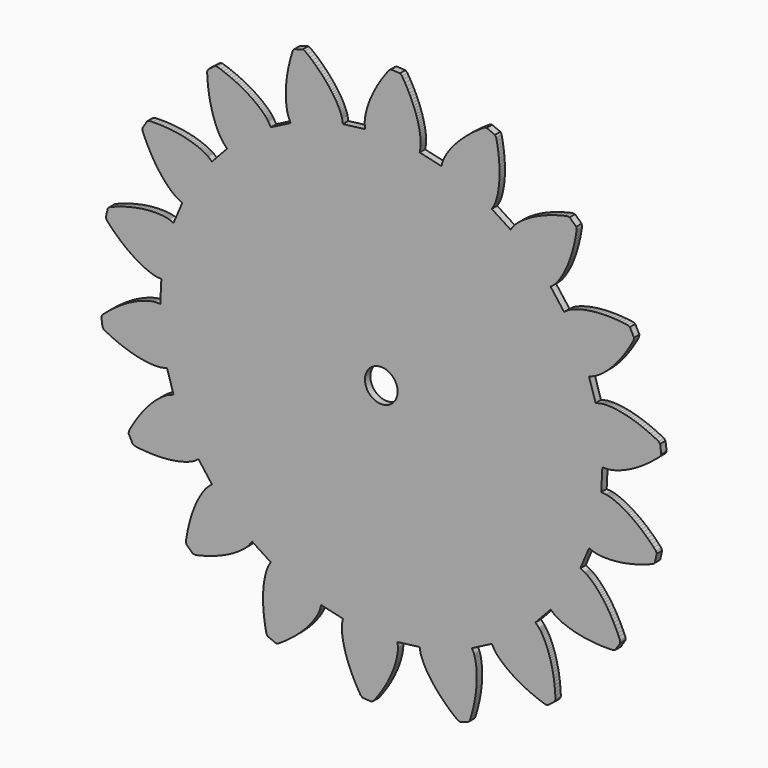
from build123d import *

# Parameters (mm, degrees)
F0_R     = 3.8384091464
F1_DEPTH = 1.5875


# Not quite as in the source:
# - a length typed as a fraction of an inch, garbled in the dataset ("3 / 203.2 mm" for 3/8 in), is restored


with BuildPart() as f1:
    # F0 (on Front) → F1 (new body)
    with BuildSketch(Plane.XZ):
        Polygon((51.660171, -5.23113), (51.924585, 0), (53.050313, 0), (53.079269, 0.00127), (53.126259, 0.002794), (53.193569, 0.008128), (53.281961, 0.014986), (53.389403, 0.025908), (53.516149, 0.042672), (53.662199, 0.0635), (53.827553, 0.090932), (54.010941, 0.124206), (54.214903, 0.166878), (54.436899, 0.216154), (54.676421, 0.275336), (54.935755, 0.343154), (55.211091, 0.42291), (55.504715, 0.513842), (55.814849, 0.61595), (56.142763, 0.73025), (56.487187, 0.85852), (56.847105, 1.000506), (57.221755, 1.157478), (57.613169, 1.329944), (58.018299, 1.518666), (58.436891, 1.722628), (58.871231, 1.94437), (59.317763, 2.183892), (59.776487, 2.441956), (60.247911, 2.718816), (60.730003, 3.01498), (61.223525, 3.331972), (61.727969, 3.669538), (62.242065, 4.027932), (62.764035, 4.40817), (63.296165, 4.809236), (63.834899, 5.23367), (64.380491, 5.681472), (64.933449, 6.152642), (65.491487, 6.647688), (65.759965, 7.135622), (65.498091, 9.23417), (65.119377, 9.64057), (64.456437, 9.983978), (63.804419, 10.305034), (63.165355, 10.603992), (62.537975, 10.8839), (61.924819, 11.142726), (61.324109, 11.382756), (60.738385, 11.604498), (60.166631, 11.806936), (59.611387, 11.992864), (59.069605, 12.161266), (58.544587, 12.31392), (58.037603, 12.451842), (57.545605, 12.574778), (57.069863, 12.681966), (56.613933, 12.778486), (56.174259, 12.861036), (55.754143, 12.931394), (55.351553, 12.9921), (54.967505, 13.04036), (54.601999, 13.080238), (54.257575, 13.111988), (53.930931, 13.133832), (53.623591, 13.150342), (53.336825, 13.158978), (53.069871, 13.163042), (52.821459, 13.160248), (52.594383, 13.15466), (52.387627, 13.145008), (52.200175, 13.132816), (52.033297, 13.1191), (51.887247, 13.102336), (51.760755, 13.08735), (51.653059, 13.07211), (51.566191, 13.05687), (51.499897, 13.045694), (51.453415, 13.036042), (51.425475, 13.029438), (50.334291, 12.753594), (48.793781, 17.758664), (49.852199, 18.144744), (49.876837, 18.154142), (49.922303, 18.1737), (49.984533, 18.201132), (50.062765, 18.238216), (50.160809, 18.285206), (50.273585, 18.342864), (50.403125, 18.413222), (50.549175, 18.494756), (50.711735, 18.589498), (50.888265, 18.698464), (51.079781, 18.8214), (51.285013, 18.958814), (51.504215, 19.111976), (51.737133, 19.27987), (51.982497, 19.466306), (52.238783, 19.668744), (52.507515, 19.889216), (52.785899, 20.126198), (53.076475, 20.383754), (53.375687, 20.659598), (53.683027, 20.954238), (53.999765, 21.26996), (54.323615, 21.606256), (54.655847, 21.961856), (54.993413, 22.34057), (55.336313, 22.740366), (55.683785, 23.160482), (56.036591, 23.60422), (56.392191, 24.071326), (56.750331, 24.560784), (57.110249, 25.073356), (57.472453, 25.608026), (57.833641, 26.167588), (58.194575, 26.751788), (58.555509, 27.358086), (58.913903, 27.9908), (59.268233, 28.646628), (59.353577, 29.196538), (58.388885, 31.078932), (57.894093, 31.331154), (57.154191, 31.42742), (56.432069, 31.50616), (55.729505, 31.567882), (55.044213, 31.616142), (54.378987, 31.650686), (53.732557, 31.669736), (53.106955, 31.678372), (52.500403, 31.672784), (51.913409, 31.657544), (51.348513, 31.631382), (50.802921, 31.595822), (50.277903, 31.550356), (49.774983, 31.497778), (49.291113, 31.437072), (48.829341, 31.371032), (48.388397, 31.29788), (47.968281, 31.220664), (47.570009, 31.139638), (47.192311, 31.053786), (46.835441, 30.967172), (46.500669, 30.87751), (46.186471, 30.787848), (45.892847, 30.69717), (45.619797, 30.607508), (45.368083, 30.51937), (45.134911, 30.432756), (44.924091, 30.349698), (44.732575, 30.269942), (44.560363, 30.19425), (44.408725, 30.123892), (44.276391, 30.059122), (44.162091, 30.00121), (44.066841, 29.950156), (43.991149, 29.907484), (43.931713, 29.873194), (43.891835, 29.846778), (43.868721, 29.832808), (42.937049, 29.199332), (39.777035, 33.375854), (40.639619, 34.10077), (40.660447, 34.118804), (40.694737, 34.152078), (40.744521, 34.19856), (40.806497, 34.260536), (40.880919, 34.338006), (40.967787, 34.431732), (41.066847, 34.541714), (41.175813, 34.66846), (41.294431, 34.813494), (41.423971, 34.976054), (41.561893, 35.156394), (41.707943, 35.356292), (41.862121, 35.575494), (42.021887, 35.812476), (42.188765, 36.071556), (42.360977, 36.348416), (42.538777, 36.647628), (42.719371, 36.96716), (42.903775, 37.30752), (43.089957, 37.668454), (43.278933, 38.051486), (43.468925, 38.45687), (43.659171, 38.882828), (43.847893, 39.330376), (44.035091, 39.8018), (44.221527, 40.293798), (44.404661, 40.809164), (44.583731, 41.346628), (44.758737, 41.905936), (44.928155, 42.488866), (45.090715, 43.093894), (45.246671, 43.72102), (45.395515, 44.369736), (45.535977, 45.042582), (45.666787, 45.735748), (45.786675, 46.452282), (45.897165, 47.189644), (45.788199, 47.735236), (44.237783, 49.175416), (43.686603, 49.242726), (42.958893, 49.078642), (42.253281, 48.90643), (41.571291, 48.724566), (40.911399, 48.535844), (40.274621, 48.34001), (39.659941, 48.137572), (39.070153, 47.930816), (38.501193, 47.718726), (37.955347, 47.503588), (37.432869, 47.28591), (36.932743, 47.065438), (36.454715, 46.843442), (36.000055, 46.6217), (35.565715, 46.399704), (35.154997, 46.179232), (34.765107, 45.960284), (34.397315, 45.743876), (34.051113, 45.531532), (33.724977, 45.322236), (33.420177, 45.118528), (33.134935, 44.9199), (32.870521, 44.728384), (32.624903, 44.542456), (32.399097, 44.364656), (32.192341, 44.194984), (32.005143, 44.034964), (31.833947, 43.88358), (31.682563, 43.742864), (31.546165, 43.613578), (31.427547, 43.49496), (31.325693, 43.388788), (31.238825, 43.296332), (31.165927, 43.215306), (31.109285, 43.149266), (31.066613, 43.096688), (31.036387, 43.059604), (31.019877, 43.037506), (30.361255, 42.123614), (25.962483, 44.96816), (26.525855, 45.94352), (26.538555, 45.968666), (26.560399, 46.009814), (26.590625, 46.072044), (26.627709, 46.150276), (26.671905, 46.249844), (26.721435, 46.366938), (26.775283, 46.504606), (26.834465, 46.660308), (26.897965, 46.838108), (26.962735, 47.033688), (27.031569, 47.251366), (27.100403, 47.488348), (27.169491, 47.746158), (27.239849, 48.026066), (27.307159, 48.32477), (27.374977, 48.64481), (27.437969, 48.986186), (27.500199, 49.348898), (27.556587, 49.73066), (27.607641, 50.134266), (27.654631, 50.5587), (27.694509, 51.003708), (27.726259, 51.469544), (27.750897, 51.955954), (27.767661, 52.461922), (27.773249, 52.98821), (27.768931, 53.535326), (27.753691, 54.101492), (27.726259, 54.68747), (27.686127, 55.292244), (27.632533, 55.916576), (27.564969, 56.559958), (27.482165, 57.220104), (27.384375, 57.899554), (27.270075, 58.597038), (27.137741, 59.310778), (26.988897, 60.041028), (26.701115, 60.517786), (24.750903, 61.340492), (24.209375, 61.215016), (23.582503, 60.81268), (22.978999, 60.40882), (22.398609, 60.005214), (21.843365, 59.601354), (21.312759, 59.199272), (20.804505, 58.799476), (20.320635, 58.402728), (19.858863, 58.010044), (19.419443, 57.62117), (19.003137, 57.236614), (18.607659, 56.85917), (18.235549, 56.48706), (17.882743, 56.121808), (17.552035, 55.766208), (17.240631, 55.41772), (16.950055, 55.078884), (16.677005, 54.749192), (16.425037, 54.431184), (16.189325, 54.123844), (15.972663, 53.827426), (15.773019, 53.543454), (15.589631, 53.272182), (15.423007, 53.014372), (15.271369, 52.770532), (15.136241, 52.540408), (15.013813, 52.32527), (14.904847, 52.125626), (14.809597, 51.940714), (14.727047, 51.77282), (14.655419, 51.621182), (14.596237, 51.486054), (14.546453, 51.36896), (14.506575, 51.268376), (14.474825, 51.18735), (14.452981, 51.122326), (14.437741, 51.07686), (14.429359, 51.050698), (14.122019, 49.967642), (9.016619, 51.136042), (9.212199, 52.244244), (9.216263, 52.2732), (9.222105, 52.319936), (9.230233, 52.3875), (9.237091, 52.474114), (9.245219, 52.58181), (9.251061, 52.709826), (9.256141, 52.8574), (9.257665, 53.025548), (9.256141, 53.213), (9.251061, 53.419756), (9.239631, 53.646832), (9.223375, 53.89372), (9.201277, 54.159404), (9.170797, 54.44617), (9.132443, 54.750716), (9.085453, 55.074566), (9.029065, 55.41645), (8.962771, 55.777384), (8.885809, 56.156606), (8.796147, 56.553354), (8.694293, 56.967882), (8.579485, 57.400698), (8.451469, 57.8485), (8.308213, 58.314336), (8.149971, 58.795158), (7.974457, 59.292744), (7.784465, 59.803792), (7.575169, 60.331858), (7.349109, 60.872116), (7.105269, 61.42736), (6.842125, 61.99505), (6.558153, 62.57671), (6.254877, 63.169292), (5.930011, 63.774066), (5.583809, 64.390016), (5.215763, 65.015872), (4.826127, 65.651126), (4.391787, 65.999614), (2.279269, 66.10731), (1.813687, 65.804034), (1.360043, 65.210182), (0.931799, 64.624458), (0.524891, 64.047116), (0.141859, 63.478156), (-0.220345, 62.918594), (-0.560959, 62.369954), (-0.880491, 61.83122), (-1.179703, 61.303154), (-1.459357, 60.788042), (-1.719707, 60.283598), (-1.961007, 59.794394), (-2.184019, 59.317636), (-2.390775, 58.854594), (-2.579497, 58.405522), (-2.753487, 57.972706), (-2.910459, 57.554876), (-3.053715, 57.152794), (-3.181985, 56.766714), (-3.297809, 56.397398), (-3.401187, 56.044592), (-3.490595, 55.70982), (-3.570351, 55.391558), (-3.639185, 55.0926), (-3.697097, 54.811422), (-3.746881, 54.548278), (-3.788029, 54.304438), (-3.821303, 54.079648), (-3.847465, 53.874416), (-3.868039, 53.688488), (-3.883279, 53.520086), (-3.894201, 53.374036), (-3.899789, 53.24602), (-3.903853, 53.138578), (-3.905123, 53.050186), (-3.903853, 52.982876), (-3.902329, 52.934616), (-3.901313, 52.90693), (-3.818509, 51.783742), (-9.016619, 51.136042), (-9.211945, 52.244244), (-9.217787, 52.271676), (-9.228709, 52.318666), (-9.245219, 52.384706), (-9.267317, 52.47005), (-9.296273, 52.573428), (-9.334881, 52.694586), (-9.380347, 52.835556), (-9.436735, 52.993798), (-9.501759, 53.168804), (-9.577197, 53.361844), (-9.665335, 53.570886), (-9.764903, 53.79847), (-9.877679, 54.041294), (-10.004425, 54.29885), (-10.143617, 54.571392), (-10.297795, 54.861206), (-10.468991, 55.162704), (-10.654919, 55.47995), (-10.857357, 55.809134), (-11.076559, 56.152288), (-11.313541, 56.506364), (-11.570081, 56.872886), (-11.844147, 57.250584), (-12.137517, 57.639204), (-12.451969, 58.037476), (-12.785217, 58.443876), (-13.139547, 58.860182), (-13.515467, 59.284616), (-13.912469, 59.714638), (-14.332839, 60.152788), (-14.775307, 60.596526), (-15.239619, 61.045598), (-15.727553, 61.498988), (-16.240125, 61.956442), (-16.774795, 62.416944), (-17.335881, 62.878208), (-17.920081, 63.343028), (-18.444845, 63.522098), (-20.468209, 62.899036), (-20.802981, 62.455298), (-21.024723, 61.743082), (-21.227415, 61.045598), (-21.411819, 60.363354), (-21.577173, 59.698128), (-21.726017, 59.048904), (-21.858351, 58.416444), (-21.974175, 57.800494), (-22.074759, 57.20207), (-22.161373, 56.622188), (-22.234525, 56.061356), (-22.293707, 55.517034), (-22.340697, 54.993286), (-22.375241, 54.487572), (-22.399879, 54.000908), (-22.415119, 53.535326), (-22.420707, 53.08727), (-22.416389, 52.661566), (-22.405467, 52.253642), (-22.387687, 51.867816), (-22.364319, 51.501294), (-22.333839, 51.1556), (-22.300819, 50.830226), (-22.261957, 50.52568), (-22.220809, 50.241708), (-22.178137, 49.977294), (-22.132417, 49.73447), (-22.086951, 49.511458), (-22.041485, 49.308766), (-21.997543, 49.127156), (-21.954617, 48.964342), (-21.913469, 48.82261), (-21.876385, 48.701198), (-21.843365, 48.599344), (-21.812885, 48.515016), (-21.789517, 48.45177), (-21.773007, 48.407828), (-21.761831, 48.381666), (-21.300313, 47.354744), (-25.962229, 44.96816), (-26.525601, 45.94352), (-26.539317, 45.967142), (-26.565987, 46.00702), (-26.604341, 46.063408), (-26.654125, 46.135036), (-26.717117, 46.221904), (-26.794587, 46.324266), (-26.885519, 46.439836), (-26.991691, 46.5709), (-27.114119, 46.712632), (-27.250517, 46.868334), (-27.405203, 47.034958), (-27.575891, 47.214282), (-27.764613, 47.403004), (-27.971369, 47.603156), (-28.197429, 47.810928), (-28.441269, 48.029876), (-28.704413, 48.255936), (-28.987115, 48.488854), (-29.290137, 48.730154), (-29.613987, 48.976788), (-29.958665, 49.22901), (-30.323663, 49.485042), (-30.711013, 49.74717), (-31.120207, 50.011838), (-31.550229, 50.277776), (-32.003619, 50.546254), (-32.478853, 50.81651), (-32.976439, 51.086766), (-33.497393, 51.355244), (-34.041715, 51.622706), (-34.609405, 51.888644), (-35.199193, 52.151788), (-35.813873, 52.410614), (-36.450397, 52.665884), (-37.110543, 52.915058), (-37.795327, 53.157882), (-38.503733, 53.393594), (-39.058977, 53.382164), (-40.7471626, 52.104798), (-40.9083764, 51.572922), (-40.8739594, 50.828956), (-40.8257248, 50.103786), (-40.7664666, 49.399698), (-40.694737, 48.717708), (-40.612187, 48.056292), (-40.519731, 47.41672), (-40.417877, 46.7995), (-40.308911, 46.202854), (-40.190547, 45.628306), (-40.066341, 45.075348), (-39.936801, 44.54525), (-39.801927, 44.034964), (-39.662735, 43.548554), (-39.519225, 43.082972), (-39.373175, 42.640504), (-39.224331, 42.218864), (-39.075487, 41.817798), (-38.926643, 41.440354), (-38.778053, 41.08196), (-38.629209, 40.747188), (-38.483159, 40.431466), (-38.339649, 40.137842), (-38.200457, 39.863776), (-38.064059, 39.611554), (-37.933249, 39.378636), (-37.807773, 39.165276), (-37.689409, 38.970966), (-37.577649, 38.79596), (-37.473001, 38.640004), (-37.377751, 38.50386), (-37.291137, 38.383972), (-37.213921, 38.281864), (-37.147627, 38.197536), (-37.091239, 38.128956), (-37.047043, 38.078156), (-37.015547, 38.042088), (-36.997513, 38.02126), (-36.212145, 37.213794), (-39.777035, 33.375854), (-40.639619, 34.10077), (-40.661717, 34.117534), (-40.699055, 34.146236), (-40.754046, 34.186114), (-40.8257248, 34.237422), (-40.9153106, 34.298128), (-41.0228034, 34.366708), (-41.1481778, 34.444178), (-41.29151, 34.529522), (-41.455467, 34.621978), (-41.6373564, 34.721038), (-41.8399722, 34.825686), (-42.0618158, 34.934398), (-42.3029888, 35.047682), (-42.5661836, 35.164776), (-42.848657, 35.284664), (-43.1532284, 35.405822), (-43.4770784, 35.528504), (-43.8229756, 35.651186), (-44.1908692, 35.773614), (-44.5794892, 35.895026), (-44.9887594, 36.013644), (-45.4201022, 36.130738), (-45.8734922, 36.243514), (-46.347507, 36.35121), (-46.8436198, 36.454588), (-47.3617544, 36.552378), (-47.9005392, 36.64331), (-48.4600504, 36.72586), (-49.0415834, 36.801806), (-49.6451636, 36.866576), (-50.2694194, 36.922964), (-50.9129538, 36.96716), (-51.5785354, 37.001704), (-52.2647926, 37.022278), (-52.9703538, 37.03066), (-53.6965906, 37.025072), (-54.442106, 37.004498), (-54.9616376, 36.803076), (-56.1109114, 35.026854), (-56.0805838, 34.47161), (-55.7939448, 33.784032), (-55.5004478, 33.118298), (-55.2041822, 32.478726), (-54.9023794, 31.861506), (-54.599205, 31.269178), (-54.293262, 30.698694), (-53.9873698, 30.152848), (-53.6800806, 29.63037), (-53.372766, 29.130244), (-53.0668484, 28.653486), (-52.7636486, 28.198826), (-52.4618458, 27.767534), (-52.1642086, 27.356816), (-51.8707116, 26.967942), (-51.5826756, 26.60142), (-51.2988306, 26.255726), (-51.0218182, 25.931876), (-50.75174, 25.62733), (-50.4898914, 25.342088), (-50.2363232, 25.07742), (-49.9910354, 24.830786), (-49.755425, 24.603456), (-49.530762, 24.395176), (-49.3171988, 24.20366), (-49.1146338, 24.028654), (-48.923067, 23.871682), (-48.7453178, 23.72995), (-48.5799384, 23.60422), (-48.4297228, 23.494238), (-48.2919278, 23.397464), (-48.1692966, 23.314914), (-48.0631754, 23.24481), (-47.9708464, 23.187914), (-47.8950528, 23.143972), (-47.8371916, 23.109682), (-47.7944688, 23.087584), (-47.7696784, 23.075138), (-46.755431, 22.584664), (-48.793527, 17.758664), (-49.8518688, 18.144744), (-49.8780308, 18.152872), (-49.9235222, 18.167858), (-49.9882922, 18.185892), (-50.0737378, 18.20926), (-50.178462, 18.235422), (-50.3024648, 18.263108), (-50.4471686, 18.29308), (-50.611151, 18.325084), (-50.797206, 18.35531), (-51.0011426, 18.385536), (-51.2271264, 18.414492), (-51.4738366, 18.442178), (-51.7398, 18.4658), (-52.0264136, 18.48612), (-52.3323312, 18.50136), (-52.660296, 18.511266), (-53.0061932, 18.515076), (-53.3741376, 18.512536), (-53.7613606, 18.50136), (-54.1678876, 18.483834), (-54.5936932, 18.454878), (-55.0388028, 18.416016), (-55.503191, 18.367756), (-55.9855116, 18.307304), (-56.4871108, 18.235422), (-57.006617, 18.150078), (-57.544081, 18.050764), (-58.0994266, 17.936464), (-58.6713076, 17.808194), (-59.2597494, 17.663414), (-59.8660728, 17.502378), (-60.4861884, 17.324578), (-61.124211, 17.128998), (-61.7760512, 16.91386), (-62.4416328, 16.679672), (-63.1223782, 16.426434), (-63.8155188, 16.15186), (-64.234441, 15.786608), (-64.7071096, 13.72362), (-64.4893808, 13.212572), (-63.9836414, 12.663932), (-63.4806706, 12.138914), (-62.9831862, 11.638788), (-62.489842, 11.162284), (-62.0006634, 10.708386), (-61.5197144, 10.277348), (-61.0443026, 9.869678), (-60.5771204, 9.483598), (-60.1168978, 9.1186), (-59.6676226, 8.775192), (-59.2266532, 8.451342), (-58.7953612, 8.149844), (-58.375042, 7.865872), (-57.9671434, 7.601204), (-57.5702684, 7.356094), (-57.1857886, 7.126986), (-56.8137294, 6.916166), (-56.4568086, 6.723634), (-56.1123084, 6.54558), (-55.7829466, 6.38302), (-55.4687486, 6.2357), (-55.171086, 6.103366), (-54.8872156, 5.983478), (-54.6212522, 5.875782), (-54.3704526, 5.78231), (-54.13756, 5.699506), (-53.9225998, 5.627878), (-53.724175, 5.565648), (-53.5436064, 5.513578), (-53.3823926, 5.469382), (-53.2391112, 5.433314), (-53.1150576, 5.404358), (-53.0089364, 5.382514), (-52.9221192, 5.366004), (-52.8559776, 5.355082), (-52.80914, 5.34797), (-52.7802094, 5.345176), (-51.6598408, 5.230876), (-51.9244326, 0), (-53.0502876, 0), (-53.0792182, -0.001524), (-53.1260812, -0.002794), (-53.1936198, -0.008128), (-53.2818086, -0.01524), (-53.389276, -0.026162), (-53.5160728, -0.042672), (-53.6621482, -0.0635), (-53.8275022, -0.091186), (-54.0107886, -0.124206), (-54.2147506, -0.166878), (-54.4365942, -0.216408), (-54.6763956, -0.27559), (-54.9354756, -0.343408), (-55.2110656, -0.423164), (-55.5045626, -0.514096), (-55.8146204, -0.61595), (-56.1426106, -0.73025), (-56.4871108, -0.858774), (-56.8467748, -1.000506), (-57.2216026, -1.157478), (-57.6129658, -1.329944), (-58.0180958, -1.518666), (-58.4370434, -1.722628), (-58.8711294, -1.944624), (-59.3176106, -2.184146), (-59.776487, -2.441956), (-60.2477586, -2.718816), (-60.7300792, -3.015234), (-61.2234488, -3.331972), (-61.7278166, -3.669792), (-62.241811, -4.028186), (-62.7640858, -4.408424), (-63.2960126, -4.80949), (-63.8348228, -5.233924), (-64.3805164, -5.681472), (-64.9331188, -6.152896), (-65.491233, -6.647942), (-65.7599396, -7.135622), (-65.4981164, -9.234424), (-65.1191484, -9.640824), (-64.45631, -9.983978), (-63.8044952, -10.305034), (-63.165101, -10.604246), (-62.5380766, -10.8839), (-61.9248698, -11.14298), (-61.3240328, -11.382756), (-60.738385, -11.604752), (-60.1664786, -11.80719), (-59.6111584, -11.993118), (-59.0695542, -12.16152), (-58.5445362, -12.314174), (-58.0373998, -12.452096), (-57.5454526, -12.574778), (-57.0700154, -12.68222), (-56.6139076, -12.77874), (-56.1743098, -12.86129), (-55.754016, -12.931394), (-55.3516038, -12.9921), (-54.9671494, -13.040614), (-54.6019482, -13.080492), (-54.2574734, -13.112242), (-53.9308548, -13.134086), (-53.6235656, -13.150596), (-53.3369266, -13.158978), (-53.0695916, -13.163042), (-52.8215606, -13.160502), (-52.5941544, -13.154914), (-52.3874492, -13.145262), (-52.2000226, -13.13307), (-52.033297, -13.118846), (-51.8872216, -13.10259), (-51.7604756, -13.08735), (-51.6529828, -13.072364), (-51.5661656, -13.057124), (-51.4999986, -13.045694), (-51.453161, -13.036296), (-51.4255766, -13.029692), (-50.3341894, -12.753594), (-48.793527, -17.758918), (-49.8518688, -18.144744), (-49.8766592, -18.154396), (-49.9221506, -18.1737), (-49.984152, -18.201386), (-50.0627142, -18.23847), (-50.160555, -18.285206), (-50.2735342, -18.343118), (-50.4030742, -18.413222), (-50.549175, -18.494756), (-50.7117604, -18.589752), (-50.8881634, -18.698718), (-51.0797048, -18.8214), (-51.2850384, -18.959068), (-51.5041388, -19.11223), (-51.737006, -19.280124), (-51.9823192, -19.466306), (-52.2386306, -19.668744), (-52.5073372, -19.889216), (-52.7856958, -20.126452), (-53.076475, -20.384008), (-53.3755092, -20.659344), (-53.6828238, -20.954492), (-53.999765, -21.270214), (-54.323615, -21.606256), (-54.65572, -21.961856), (-54.9933114, -22.340824), (-55.3364654, -22.740366), (-55.6837088, -23.160736), (-56.0364894, -23.604474), (-56.3920386, -24.07158), (-56.750331, -24.560784), (-57.109995, -25.073356), (-57.4724276, -25.60828), (-57.8334632, -26.167842), (-58.1944988, -26.752042), (-58.5555598, -27.35834), (-58.9138522, -27.9908), (-59.2680044, -28.646628), (-59.35345, -29.196792), (-58.3888088, -31.078932), (-57.8941184, -31.331154), (-57.1540894, -31.427674), (-56.4319928, -31.50616), (-55.7292256, -31.568136), (-55.0442892, -31.616396), (-54.3787076, -31.65094), (-53.73243, -31.670244), (-53.1068026, -31.678372), (-52.5004538, -31.672784), (-51.9133836, -31.657798), (-51.3484114, -31.631636), (-50.8027178, -31.595822), (-50.2776744, -31.550356), (-49.7746782, -31.498032), (-49.2910114, -31.437326), (-48.8293664, -31.371032), (-48.388397, -31.298134), (-47.9681032, -31.220918), (-47.5698312, -31.139638), (-47.1922348, -31.05404), (-46.8353394, -30.967426), (-46.5004658, -30.877764), (-46.1862932, -30.788102), (-45.8927454, -30.697424), (-45.6198986, -30.607762), (-45.3677528, -30.519624), (-45.1348348, -30.432756), (-44.9239894, -30.349952), (-44.7324734, -30.270196), (-44.5602106, -30.19425), (-44.4086234, -30.124146), (-44.2763148, -30.059122), (-44.1619386, -30.001464), (-44.0668664, -29.950156), (-43.9910728, -29.907484), (-43.9317892, -29.873194), (-43.8918604, -29.846778), (-43.8684416, -29.833062), (-42.9368458, -29.199586), (-39.777035, -33.376108), (-40.639619, -34.101024), (-40.660447, -34.118804), (-40.694737, -34.152078), (-40.744521, -34.198814), (-40.8064208, -34.26079), (-40.8808428, -34.338006), (-40.96766, -34.431732), (-41.0668978, -34.541968), (-41.1757114, -34.668714), (-41.2942532, -34.813494), (-41.4237932, -34.976054), (-41.5615882, -35.156648), (-41.7076636, -35.356546), (-41.8620194, -35.575494), (-42.0218616, -35.812476), (-42.1885872, -36.071556), (-42.36085, -36.34867), (-42.5385992, -36.647628), (-42.719117, -36.967414), (-42.9038004, -37.307774), (-43.08983, -37.668708), (-43.2786282, -38.05174), (-43.4687726, -38.45687), (-43.6589678, -38.882828), (-43.847766, -39.33063), (-44.0351672, -39.802054), (-44.2212222, -40.293798), (-44.4044832, -40.8093164), (-44.5836294, -41.3467296), (-44.7586354, -41.9062408), (-44.928155, -42.4891454), (-45.0907404, -43.0940718), (-45.2464678, -43.7210962), (-45.3952864, -44.3701424), (-45.53585, -45.0426328), (-45.6667616, -45.7357734), (-45.786675, -46.4523836), (-45.896911, -47.1896186), (-45.7880466, -47.7353376), (-44.2377322, -49.1753652), (-43.6865014, -49.2428784), (-42.9589184, -49.0789214), (-42.2533572, -48.9066586), (-41.5712148, -48.7247692), (-40.911145, -48.5359456), (-40.274621, -48.340264), (-39.659941, -48.137699), (-39.070153, -47.9310192), (-38.500939, -47.7187768), (-37.955347, -47.5037912), (-37.432869, -47.2861132), (-36.932743, -47.0656158), (-36.454461, -46.8437468), (-35.999801, -46.6218524), (-35.565715, -46.3999834), (-35.154997, -46.1795114), (-34.765107, -45.9603856), (-34.397061, -45.7440792), (-34.051367, -45.5318368), (-33.724723, -45.3223884), (-33.420177, -45.1184264), (-33.134935, -44.9199762), (-32.870267, -44.7284602), (-32.624903, -44.5424052), (-32.399097, -44.3646306), (-32.192341, -44.1951364), (-32.004889, -44.0352942), (-31.833947, -43.883707), (-31.682563, -43.7431434), (-31.545911, -43.6136034), (-31.427547, -43.4951124), (-31.325439, -43.3889912), (-31.238825, -43.2966876), (-31.165673, -43.2153568), (-31.109285, -43.1492152), (-31.066359, -43.0968658), (-31.036133, -43.0596548), (-31.019623, -43.0376076), (-30.360747, -42.1239442), (-25.962229, -44.9682108), (-26.525601, -45.9438756), (-26.538301, -45.9686914), (-26.560145, -46.0100426), (-26.590625, -46.072044), (-26.627709, -46.1505808), (-26.671651, -46.2498186), (-26.721435, -46.366938), (-26.775029, -46.504733), (-26.834465, -46.6604604), (-26.897965, -46.8382096), (-26.962735, -47.0338912), (-27.031569, -47.2516454), (-27.100403, -47.4886528), (-27.169491, -47.7463358), (-27.239595, -48.0260914), (-27.307159, -48.3251256), (-27.374723, -48.6448354), (-27.437969, -48.9865924), (-27.499945, -49.3489996), (-27.556587, -49.7307108), (-27.607641, -50.1344946), (-27.654631, -50.5589286), (-27.694509, -51.0040128), (-27.726259, -51.469798), (-27.750897, -51.9562334), (-27.767407, -52.4619728), (-27.772995, -52.9883878), (-27.768931, -53.5354784), (-27.753691, -54.101873), (-27.726259, -54.6875208), (-27.685873, -55.292498), (-27.632279, -55.9167284), (-27.564969, -56.5602882), (-27.482165, -57.220358), (-27.384375, -57.8997318), (-27.270075, -58.597038), (-27.137741, -59.3108542), (-26.988897, -60.0412058), (-26.700607, -60.5180146), (-24.750903, -61.3406952), (-24.209375, -61.2152954), (-23.582503, -60.8129086), (-22.978745, -60.4091502), (-22.398609, -60.0053664), (-21.843365, -59.601608), (-21.312759, -59.1992212), (-20.804251, -58.799603), (-20.320635, -58.402728), (-19.858863, -58.0099678), (-19.419189, -57.6213478), (-19.003137, -57.2368934), (-18.607659, -56.8593224), (-18.235295, -56.4872378), (-17.882489, -56.122062), (-17.552035, -55.7665128), (-17.240631, -55.4178724), (-16.949801, -55.078884), (-16.676751, -54.7495476), (-16.425037, -54.4312348), (-16.189325, -54.1239202), (-15.972663, -53.8276292), (-15.773019, -53.5437334), (-15.589631, -53.2722836), (-15.423007, -53.0145752), (-15.271369, -52.770659), (-15.136241, -52.5405604), (-15.013813, -52.3255748), (-14.904847, -52.125753), (-14.809597, -51.9411204), (-14.727047, -51.7729724), (-14.655419, -51.6213852), (-14.596237, -51.4863334), (-14.546453, -51.369214), (-14.506575, -51.2686046), (-14.474825, -51.1873246), (-14.452981, -51.1225546), (-14.437741, -51.0770886), (-14.429359, -51.0508758), (-14.122019, -49.9677436), (-9.016619, -51.1363214), (-9.211945, -52.244244), (-9.216263, -52.2732254), (-9.221851, -52.320063), (-9.229979, -52.3875762), (-9.237091, -52.4743934), (-9.245219, -52.5818862), (-9.250807, -52.7100546), (-9.256141, -52.8574762), (-9.257665, -53.0256242), (-9.256141, -53.2130254), (-9.250807, -53.4197306), (-9.239631, -53.6471114), (-9.223375, -53.8937708), (-9.201023, -54.1597342), (-9.170797, -54.4463478), (-9.132189, -54.7509192), (-9.085453, -55.0747692), (-9.029065, -55.4165008), (-8.962517, -55.7775618), (-8.885301, -56.1565298), (-8.796147, -56.5534048), (-8.694293, -56.9681868), (-8.579485, -57.4008758), (-8.451469, -57.848754), (-8.308213, -58.3145392), (-8.149717, -58.7954882), (-7.974457, -59.2929218), (-7.784465, -59.804173), (-7.575169, -60.3319596), (-7.349109, -60.8721668), (-7.105269, -61.4275124), (-6.842125, -61.9952786), (-6.558153, -62.5767862), (-6.254623, -63.1693428), (-5.929757, -63.77432), (-5.583809, -64.3902954), (-5.215763, -65.0159228), (-4.825873, -65.6512022), (-4.391787, -65.9998426), (-2.279269, -66.1073354), (-1.813687, -65.804161), (-1.359789, -65.2102328), (-0.931545, -64.6245596), (-0.524891, -64.0471668), (-0.141859, -63.478029), (0.220599, -62.9185432), (0.560959, -62.3701064), (0.880491, -61.8312708), (1.179703, -61.3034842), (1.459357, -60.7880928), (1.719961, -60.2837504), (1.961261, -59.7945464), (2.184019, -59.3177376), (2.390775, -58.8546956), (2.580005, -58.4054712), (2.753487, -57.9727568), (2.910459, -57.5552062), (3.053715, -57.1528448), (3.181985, -56.7669934), (3.297809, -56.3976774), (3.401187, -56.0448968), (3.490849, -55.7100486), (3.570605, -55.3917104), (3.639185, -55.0926762), (3.697097, -54.811549), (3.746881, -54.5483542), (3.788283, -54.304438), (3.821303, -54.0798258), (3.847465, -53.8744668), (3.868293, -53.6884626), (3.883533, -53.5203146), (3.894455, -53.3742646), (3.900043, -53.2460962), (3.903853, -53.1386034), (3.905377, -53.0504146), (3.903853, -52.9829014), (3.902837, -52.9346668), (3.901313, -52.9071078), (3.818509, -51.7840214), (9.016619, -51.1363214), (9.212199, -52.244244), (9.217787, -52.2718284), (9.228709, -52.3186914), (9.245219, -52.384833), (9.267571, -52.4702786), (9.296527, -52.5736058), (9.334881, -52.6948908), (9.380347, -52.835429), (9.436735, -52.9938996), (9.501759, -53.1689056), (9.577197, -53.361844), (9.665335, -53.5713178), (9.764903, -53.7986986), (9.877933, -54.0412178), (10.004425, -54.2989262), (10.143871, -54.571773), (10.298049, -54.8611552), (10.468991, -55.162958), (10.654919, -55.4798992), (10.857357, -55.8092356), (11.076559, -56.1523896), (11.313541, -56.5065418), (11.570081, -56.8730892), (11.844147, -57.2506856), (12.137771, -57.6392802), (12.451969, -58.0375268), (12.785471, -58.4440792), (13.139547, -58.8602328), (13.515975, -59.2846668), (13.912977, -59.7146126), (14.333093, -60.1528134), (14.775307, -60.5965514), (15.239619, -61.0458012), (15.727553, -61.4991658), (16.240125, -61.9566706), (16.775049, -62.416944), (17.335881, -62.878589), (17.920081, -63.3429772), (18.445099, -63.5221234), (20.468209, -62.8992646), (20.802981, -62.455552), (21.024977, -61.743082), (21.227415, -61.0458012), (21.411819, -60.3636842), (21.577427, -59.6981026), (21.726271, -59.0490056), (21.858605, -58.4164948), (21.974175, -57.800494), (22.074759, -57.2024256), (22.161627, -56.6222896), (22.234525, -56.0614576), (22.293961, -55.5171102), (22.340697, -54.9934384), (22.375241, -54.487699), (22.400133, -54.0012636), (22.415119, -53.5354784), (22.420707, -53.0876256), (22.416643, -52.6617946), (22.405721, -52.2539214), (22.387687, -51.8680446), (22.364319, -51.5015226), (22.334093, -51.1556254), (22.300819, -50.8303784), (22.261957, -50.5258578), (22.220809, -50.2419874), (22.178137, -49.9773956), (22.132671, -49.7348764), (22.087205, -49.5116358), (22.041485, -49.3090454), (21.997543, -49.1271306), (21.954871, -48.9645452), (21.913469, -48.8225846), (21.876385, -48.7013504), (21.843365, -48.599344), (21.812885, -48.5152954), (21.789771, -48.451897), (21.773007, -48.4078026), (21.762085, -48.3816152), (21.300313, -47.354998), (25.962483, -44.9682108), (26.525855, -45.9438756), (26.539571, -45.9673198), (26.565987, -46.007274), (26.604341, -46.0637636), (26.654125, -46.135417), (26.717371, -46.2222342), (26.794587, -46.3242152), (26.885519, -46.439963), (26.991691, -46.5708746), (27.114119, -46.7128352), (27.250771, -46.8685626), (27.405203, -47.0352628), (27.575891, -47.214409), (27.764613, -47.4032326), (27.971369, -47.603029), (28.197683, -47.8111058), (28.441269, -48.0302062), (28.704413, -48.2562408), (28.987115, -48.489108), (29.290137, -48.7302556), (29.613987, -48.9769404), (29.958665, -49.229137), (30.323663, -49.485423), (30.711013, -49.7472462), (31.120207, -50.011838), (31.550483, -50.2778014), (32.003619, -50.546508), (32.478853, -50.816637), (32.976693, -51.0867152), (33.497393, -51.3554218), (34.041715, -51.6227568), (34.609405, -51.8887202), (35.199193, -52.1519404), (35.814127, -52.4110204), (36.450397, -52.6659602), (37.110543, -52.9153882), (37.795581, -53.1579074), (38.503987, -53.3935686), (39.059231, -53.3825196), (40.747315, -52.1050774), (40.908605, -51.5731506), (40.874061, -50.8290068), (40.826055, -50.104167), (40.766619, -49.3999774), (40.694737, -48.7178858), (40.612187, -48.056419), (40.519731, -47.4170248), (40.417877, -46.7996524), (40.309165, -46.2029302), (40.190547, -45.6282806), (40.066341, -45.0757036), (39.937055, -44.5451484), (39.801927, -44.0352942), (39.662735, -43.5488334), (39.519225, -43.0830736), (39.373175, -42.6407326), (39.224585, -42.2190418), (39.075741, -41.818052), (38.926897, -41.4404302), (38.778053, -41.0821632), (38.629209, -40.7472896), (38.483159, -40.43172), (38.339903, -40.138096), (38.200711, -39.86403), (38.064059, -39.611808), (37.933249, -39.37889), (37.808027, -39.165276), (37.689409, -38.970966), (37.577903, -38.79596), (37.473255, -38.640258), (37.378005, -38.50386), (37.291137, -38.383972), (37.213921, -38.281864), (37.147881, -38.19779), (37.091493, -38.128956), (37.047297, -38.078156), (37.015547, -38.042088), (36.997513, -38.021514), (36.211891, -37.214048), (39.777035, -33.376108), (40.639619, -34.101024), (40.661971, -34.117534), (40.699055, -34.14649), (40.753919, -34.186368), (40.826055, -34.237422), (40.915209, -34.298128), (41.022905, -34.366962), (41.148381, -34.444178), (41.291637, -34.529522), (41.455721, -34.621978), (41.637331, -34.721038), (41.840277, -34.82594), (42.061765, -34.934652), (42.303065, -35.047682), (42.566209, -35.164776), (42.848911, -35.284664), (43.153203, -35.406076), (43.477053, -35.528758), (43.823255, -35.65144), (44.191047, -35.773868), (44.579413, -35.89528), (44.988861, -36.013644), (45.420153, -36.130992), (45.873543, -36.243768), (46.347761, -36.351464), (46.843569, -36.454588), (47.361983, -36.552632), (47.900463, -36.643564), (48.460025, -36.726114), (49.041685, -36.80206), (49.645443, -36.86683), (50.269521, -36.923218), (50.912903, -36.967414), (51.578637, -37.001704), (52.264691, -37.022532), (52.970303, -37.03066), (53.696743, -37.025326), (54.442233, -37.004498), (54.961663, -36.80333), (56.111013, -35.027108), (56.080787, -34.47161), (55.794021, -33.784032), (55.500397, -33.118552), (55.204233, -32.47898), (54.902481, -31.86176), (54.599459, -31.269178), (54.293135, -30.698694), (53.987319, -30.153102), (53.680233, -29.630624), (53.372893, -29.130244), (53.067077, -28.65374), (52.763547, -28.19908), (52.462049, -27.767534), (52.164361, -27.356816), (51.870737, -26.968196), (51.582955, -26.601674), (51.298983, -26.25598), (51.021869, -25.93213), (50.751613, -25.627584), (50.489993, -25.342342), (50.236247, -25.077674), (49.991137, -24.83104), (49.755425, -24.603456), (49.530635, -24.39543), (49.317275, -24.203914), (49.114837, -24.028908), (48.923321, -23.871936), (48.745521, -23.72995), (48.579913, -23.604474), (48.429799, -23.494492), (48.292131, -23.397718), (48.169449, -23.315168), (48.063277, -23.245064), (47.970821, -23.188168), (47.895383, -23.143972), (47.837471, -23.109936), (47.794291, -23.087584), (47.769653, -23.075392), (46.755431, -22.584918), (48.793781, -17.758918), (49.852199, -18.144744), (49.878107, -18.152872), (49.923827, -18.168112), (49.988343, -18.186146), (50.073687, -18.209514), (50.178335, -18.235422), (50.302541, -18.263362), (50.447321, -18.293334), (50.611405, -18.325084), (50.797333, -18.355564), (51.001041, -18.38579), (51.227355, -18.414746), (51.473735, -18.442178), (51.739927, -18.4658), (52.026693, -18.486374), (52.332509, -18.501614), (52.660169, -18.51152), (53.006371, -18.51533), (53.374163, -18.51279), (53.761513, -18.501614), (54.167913, -18.483834), (54.593871, -18.454624), (55.039133, -18.41627), (55.503191, -18.367756), (55.985537, -18.307558), (56.487187, -18.235422), (57.006871, -18.150078), (57.544081, -18.051018), (58.099325, -17.936718), (58.671587, -17.808194), (59.259597, -17.663668), (59.866149, -17.502378), (60.486163, -17.324578), (61.124465, -17.129252), (61.775975, -16.914114), (62.441709, -16.679672), (63.122683, -16.42618), (63.815849, -16.152114), (64.234441, -15.786862), (64.707135, -13.723874), (64.489457, -13.212572), (63.983743, -12.664186), (63.480569, -12.139168), (62.983237, -11.639042), (62.489969, -11.162284), (62.000765, -10.70864), (61.519943, -10.277602), (61.044455, -9.869678), (60.577349, -9.483852), (60.116847, -9.1186), (59.667775, -8.775446), (59.226831, -8.451596), (58.795285, -8.149844), (58.375169, -7.865872), (57.966991, -7.601458), (57.570243, -7.356094), (57.185941, -7.12724), (56.813831, -6.916166), (56.456961, -6.723634), (56.112537, -6.545834), (55.783099, -6.383274), (55.468647, -6.2357), (55.171213, -6.103366), (54.887241, -5.983478), (54.621303, -5.876036), (54.370605, -5.782564), (54.137687, -5.699506), (53.922803, -5.627878), (53.724175, -5.565902), (53.543581, -5.513578), (53.382291, -5.469636), (53.239035, -5.433568), (53.115337, -5.404612), (53.009165, -5.382768), (52.922297, -5.366258), (52.856003, -5.355336), (52.809013, -5.348224), (52.780311, -5.34543), align=None)
        Circle(F0_R, mode=Mode.SUBTRACT)
    extrude(amount=F1_DEPTH)


solid = f1.part
